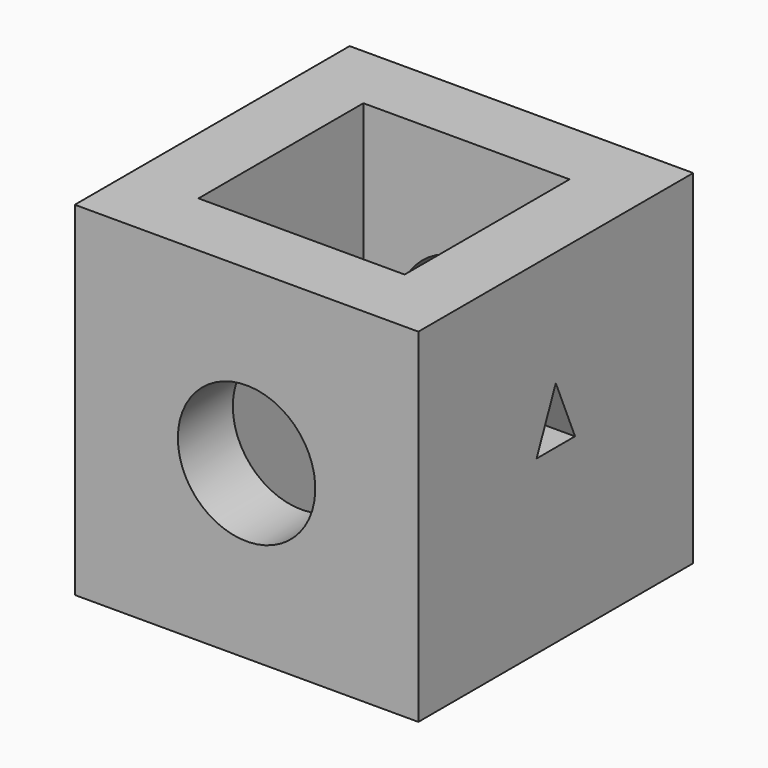
from build123d import *

# Parameters (mm, degrees)
F1_W     = 127
F1_H     = 127
F2_DEPTH = 63.5
F3_W     = 76.2
F3_H     = 76.2
F4_DEPTH = 135.636
F6_DEPTH = 146.304
F7_R     = 25.4
F8_DEPTH = 141.986


# Not quite as in the source:
# - a variable given as a bare number and used for a length is read in inches; the dataset says mm whatever the document's units were


with BuildPart() as f2:
    # F1 (on Front) → F2 (new body, symmetric)
    with BuildSketch(Plane.XZ):
        Rectangle(F1_W, F1_H)
    extrude(amount=F2_DEPTH, both=True)

    # F3 (on face) → F4 (cut)
    with BuildSketch(Plane(origin=(0, 0, -63.5), x_dir=(1, 0, 0), z_dir=(0, 0, -1))):
        Rectangle(F3_W, F3_H)
    extrude(amount=-F4_DEPTH, mode=Mode.SUBTRACT)

    # F5 (on face) → F6 (cut)
    with BuildSketch(Plane.YZ.offset(63.5)):
        Polygon((8.8900011033, 0), (0, 20.9176484495), (-8.8900011033, 0), align=None)
    extrude(amount=-F6_DEPTH, mode=Mode.SUBTRACT)

    # F7 (on face) → F8 (cut)
    with BuildSketch(Plane(origin=(0, 63.5, 0), x_dir=(-1, 0, 0), z_dir=(0, 1, 0))):
        Circle(F7_R)
    extrude(amount=-F8_DEPTH, mode=Mode.SUBTRACT)


solid = f2.part
